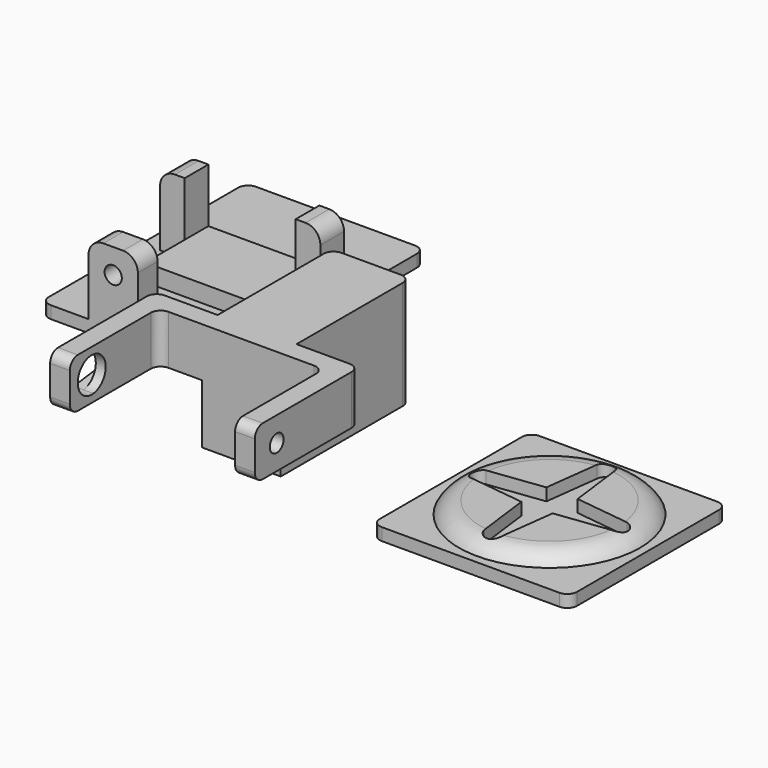
from build123d import *

# Parameters (mm, degrees)
F0_W      = 16
F0_H      = 32.9
F0_R      = 1
F0_W_2    = 12
F0_H_2    = 22.5
F1_DEPTH  = 20
F2_DEPTH  = 4
F3_W      = 16
F3_H      = 32.9
F4_DEPTH  = 2
F6_DEPTH  = 10
F7_R      = 2
F9_DEPTH  = 2
F10_DEPTH = 4
F11_W     = 40
F11_H     = 40
F12_DEPTH = 2.5
F13_W     = 5
F13_H     = 6
F13_W_2   = 10
F13_H_2   = 5
F14_DEPTH = 14.5
F15_DEPTH = 3.5
F16_R     = 3
F17_DEPTH = 12
F18_DEPTH = 3.75
F19_R     = 1.75
F20_DEPTH = 4
F21_R     = 1.75
F22_DEPTH = 5
F23_W     = 40
F23_H     = 40
F24_DEPTH = 2.5
F25_R     = 18.365
F26_DEPTH = 2.5
F28_R     = 2
F29_R     = 2


# Not quite as in the source:
# - a fillet or chamfer that OpenCascade refuses, or shapes differently, is made with other operations: its cross-section is extruded or revolved along the edge and cut away or added


with BuildPart() as f1:
    # F0 (on Top) → F1 (new body)
    with BuildSketch(Plane.XY):
        Rectangle(F0_W, F0_H)
        with Locations((0, -13.85)):
            Circle(F0_R, mode=Mode.SUBTRACT)
        Rectangle(F0_W_2, F0_H_2, mode=Mode.SUBTRACT)
        with Locations((0, 13.85)):
            Circle(F0_R, mode=Mode.SUBTRACT)
        with Locations((0, 13.85)):
            Circle(F0_R)
        with Locations((0, -13.85)):
            Circle(F0_R)
    extrude(amount=F1_DEPTH)

    # F0 (on Top) → F2 (cut)
    with BuildSketch(Plane.XY):
        with Locations((0, 13.85)):
            Circle(F0_R)
        with Locations((0, -13.85)):
            Circle(F0_R)
    extrude(amount=F2_DEPTH, mode=Mode.SUBTRACT)

    # F3 (on face) → F4 (join)
    with BuildSketch(Plane.XY.offset(20)):
        Rectangle(F3_W, F3_H)
    extrude(amount=F4_DEPTH)

    # F5 (on face) → F6 (join)
    with BuildSketch(Plane.XY.offset(22)):
        Polygon((8, -12.45), (8, -16.45), (16.75, -16.45), (16.75, -38.95), (20.75, -38.95), (20.75, -12.45), align=None)
        Polygon((-16.75, -38.95), (-16.75, -16.45), (-8, -16.45), (-8, -12.45), (-20.75, -12.45), (-20.75, -38.95), align=None)
    extrude(amount=-F6_DEPTH)

    # F7
    f7_edges = [f1.edges().sort_by_distance(p)[0] for p in [
        (-20.75, -12.45, 17),
        (20.75, -12.45, 17),
        (18.75, -38.95, 22),
        (18.75, -38.95, 12),
        (-18.75, -38.95, 22),
        (-18.75, -38.95, 12),
        (-16.75, -16.45, 17),
        (16.75, -16.45, 17),
        (-8, 16.45, 11),
        (8, 16.45, 11),
    ]]
    fillet(f7_edges, radius=F7_R)

    # F8 (on face) → F9 (cut)
    with BuildSketch(Plane(origin=(-20.75, 0, 0), x_dir=(0, -1, 0), z_dir=(-1, 0, 0))):
        with BuildLine():
            ThreePointArc((21.11, 17), (20.5076279836, 18.3347630248), (19.1082108626, 18.7661284151))
            ThreePointArc((19.1082108626, 18.7661284151), (17.55, 17), (19.1082108626, 15.2338715849))
            ThreePointArc((19.1082108626, 15.2338715849), (20.5076279836, 15.6652369752), (21.11, 17))
        make_face()
        with BuildLine():
            ThreePointArc((32.9745367412, 13.4925483442), (29.88, 17), (32.9745367412, 20.5074516558))
            Line((32.9745367412, 20.5074516558), (19.1082108626, 18.7661284151))
            ThreePointArc((19.1082108626, 18.7661284151), (20.5076279836, 18.3347630248), (21.11, 17))
            ThreePointArc((21.11, 17), (20.5076279836, 15.6652369752), (19.1082108626, 15.2338715849))
            Line((19.1082108626, 15.2338715849), (32.9745367412, 13.4925483442))
        make_face()
        with BuildLine():
            ThreePointArc((32.9745367412, 13.4925483442), (35.7537162483, 14.3492206222), (36.95, 17))
            ThreePointArc((36.95, 17), (35.7537162483, 19.6507793778), (32.9745367412, 20.5074516558))
            ThreePointArc((32.9745367412, 20.5074516558), (29.88, 17), (32.9745367412, 13.4925483442))
        make_face()
    extrude(amount=-F9_DEPTH, mode=Mode.SUBTRACT)

    # F8 (on face) → F10 (cut, through all)
    with BuildSketch(Plane(origin=(-20.75, 0, 0), x_dir=(0, -1, 0), z_dir=(-1, 0, 0))):
        with BuildLine():
            ThreePointArc((32.9745367412, 13.4925483442), (35.7537162483, 14.3492206222), (36.95, 17))
            ThreePointArc((36.95, 17), (35.7537162483, 19.6507793778), (32.9745367412, 20.5074516558))
            ThreePointArc((32.9745367412, 20.5074516558), (29.88, 17), (32.9745367412, 13.4925483442))
        make_face()
    extrude(amount=-F10_DEPTH, mode=Mode.SUBTRACT)

    # F19 (on face) → F20 (cut, through all)
    with BuildSketch(Plane(origin=(16.75, 0, 0), x_dir=(0, -1, 0), z_dir=(-1, 0, 0))):
        with Locations((33.415, 17)):
            Circle(F19_R)
    extrude(amount=-F20_DEPTH, mode=Mode.SUBTRACT)


with BuildPart() as f12:
    # F11 (on Top) → F12 (new body)
    with BuildSketch(Plane.XY):
        with Locations((-36.1275146902, 22.9365597665)):
            Rectangle(F11_W, F11_H)
    extrude(amount=F12_DEPTH)

    # F13 (on face) → F14 (join)
    with BuildSketch(Plane.XY.offset(2.5)):
        with Locations((-49.8775146902, 31.4365597665)):
            Rectangle(F13_W, F13_H)
        with Locations((-22.3775146902, 31.4365597665)):
            Rectangle(F13_W, F13_H)
        with Locations((-41.4775146902, 5.4365597665)):
            Rectangle(F13_W_2, F13_H_2)
    extrude(amount=F14_DEPTH)

    # F13 (on face) → F15 (join)
    with BuildSketch(Plane.XY.offset(2.5)):
        Polygon((-24.8775146902, 34.4365597665), (-47.3775146902, 34.4365597665), (-47.3775146902, 28.4365597665), (-47.3775146902, 18.4365597665), (-24.8775146902, 18.4365597665), (-24.8775146902, 28.4365597665), align=None)
    extrude(amount=F15_DEPTH)

    # F16
    f16_edges = [f12.edges().sort_by_distance(p)[0] for p in [
        (-52.377515, 31.43656, 17),
        (-19.877515, 31.43656, 17),
        (-46.477515, 5.43656, 17),
        (-36.477515, 5.43656, 17),
    ]]
    fillet(f16_edges, radius=F16_R)

    # F17 (add): a face of the model
    f17_faces = [f12.faces().sort_by_distance(p)[0] for p in [
        (-36.1275146902, 42.9365597665, 1.25),
    ]]
    extrude(f17_faces, amount=F17_DEPTH)

    # F18 (cut, through all): a face of the model
    f18_faces = [f12.faces().sort_by_distance(p)[0] for p in [
        (-16.1275146902, 28.9365597665, 1.25),
    ]]
    extrude(f18_faces, amount=-F18_DEPTH, mode=Mode.SUBTRACT)

    # F21 (on face) → F22 (cut, through all)
    with BuildSketch(Plane(origin=(0, 7.9365597665, 0), x_dir=(-1, 0, 0), z_dir=(0, 1, 0))):
        with Locations((41.4775146902, 12)):
            Circle(F21_R)
    extrude(amount=-F22_DEPTH, mode=Mode.SUBTRACT)

    # F29
    f29_edges = [f12.edges().sort_by_distance(p)[0] for p in [
        (-56.127515, 2.93656, 1.25),
        (-19.877515, 2.93656, 1.25),
        (-19.877515, 54.93656, 1.25),
        (-56.127515, 54.93656, 1.25),
    ]]
    fillet(f29_edges, radius=F29_R)


with BuildPart() as f24:
    # F23 (on Top) → F24 (new body)
    with BuildSketch(Plane.XY):
        with Locations((49.3299849331, 0)):
            Rectangle(F23_W, F23_H)
        with BuildLine():
            ThreePointArc((35.0231957958, -1.7661284151), (33.4649849331, 0), (35.0231957958, 1.7661284151))
            Line((35.0231957958, 1.7661284151), (46.164712816, 3.1652721172))
            Line((46.164712816, 3.1652721172), (47.5638565181, 14.3067891374))
            ThreePointArc((47.5638565181, 14.3067891374), (49.3299849331, 15.865), (51.0961133482, 14.3067891374))
            Line((51.0961133482, 14.3067891374), (52.4952570503, 3.1652721172))
            Line((52.4952570503, 3.1652721172), (63.6367740705, 1.7661284151))
            ThreePointArc((63.6367740705, 1.7661284151), (64.7497479579, 1.1776279836), (65.1949849331, 0))
            ThreePointArc((65.1949849331, 0), (64.7497479579, -1.1776279836), (63.6367740705, -1.7661284151))
            Line((63.6367740705, -1.7661284151), (52.4952570503, -3.1652721172))
            Line((52.4952570503, -3.1652721172), (51.0961133482, -14.3067891374))
            ThreePointArc((51.0961133482, -14.3067891374), (49.3299849331, -15.865), (47.5638565181, -14.3067891374))
            Line((47.5638565181, -14.3067891374), (46.164712816, -3.1652721172))
            Line((46.164712816, -3.1652721172), (35.0231957958, -1.7661284151))
        make_face(mode=Mode.SUBTRACT)
        with BuildLine():
            ThreePointArc((35.0231957958, 1.7661284151), (36.4226129167, 1.3347630248), (37.0249849331, 0))
            ThreePointArc((37.0249849331, 0), (36.4226129167, -1.3347630248), (35.0231957958, -1.7661284151))
            Line((35.0231957958, -1.7661284151), (46.164712816, -3.1652721172))
            Line((46.164712816, -3.1652721172), (47.5638565181, -14.3067891374))
            ThreePointArc((47.5638565181, -14.3067891374), (49.21887368, -12.308471281), (51.1099849331, -14.085))
            ThreePointArc((51.1099849331, -14.085), (51.1065136521, -14.1961112532), (51.0961133482, -14.3067891374))
            Line((51.0961133482, -14.3067891374), (52.4952570503, -3.1652721172))
            Line((52.4952570503, -3.1652721172), (63.6367740705, -1.7661284151))
            ThreePointArc((63.6367740705, -1.7661284151), (61.6349849331, 0), (63.6367740705, 1.7661284151))
            Line((63.6367740705, 1.7661284151), (52.4952570503, 3.1652721172))
            Line((52.4952570503, 3.1652721172), (51.0961133482, 14.3067891374))
            ThreePointArc((51.0961133482, 14.3067891374), (51.1065136521, 14.1961112532), (51.1099849331, 14.085))
            ThreePointArc((51.1099849331, 14.085), (49.21887368, 12.308471281), (47.5638565181, 14.3067891374))
            Line((47.5638565181, 14.3067891374), (46.164712816, 3.1652721172))
            Line((46.164712816, 3.1652721172), (35.0231957958, 1.7661284151))
        make_face()
        with BuildLine():
            ThreePointArc((51.0961133482, 14.3067891374), (49.3299849331, 15.865), (47.5638565181, 14.3067891374))
            ThreePointArc((47.5638565181, 14.3067891374), (49.21887368, 12.308471281), (51.1099849331, 14.085))
            ThreePointArc((51.1099849331, 14.085), (51.1065136521, 14.1961112532), (51.0961133482, 14.3067891374))
        make_face()
        with BuildLine():
            ThreePointArc((35.0231957958, -1.7661284151), (36.4226129167, -1.3347630248), (37.0249849331, 0))
            ThreePointArc((37.0249849331, 0), (36.4226129167, 1.3347630248), (35.0231957958, 1.7661284151))
            ThreePointArc((35.0231957958, 1.7661284151), (33.4649849331, 0), (35.0231957958, -1.7661284151))
        make_face()
        with BuildLine():
            ThreePointArc((51.1099849331, -14.085), (49.21887368, -12.308471281), (47.5638565181, -14.3067891374))
            ThreePointArc((47.5638565181, -14.3067891374), (49.3299849331, -15.865), (51.0961133482, -14.3067891374))
            ThreePointArc((51.0961133482, -14.3067891374), (51.1065136521, -14.1961112532), (51.1099849331, -14.085))
        make_face()
        with BuildLine():
            ThreePointArc((65.1949849331, 0), (64.7497479579, 1.1776279836), (63.6367740705, 1.7661284151))
            ThreePointArc((63.6367740705, 1.7661284151), (61.6349849331, 0), (63.6367740705, -1.7661284151))
            ThreePointArc((63.6367740705, -1.7661284151), (64.7497479579, -1.1776279836), (65.1949849331, 0))
        make_face()
    extrude(amount=-F24_DEPTH)

    # F25 (on face) → F26 (join)
    with BuildSketch(Plane.XY):
        with Locations((49.3299849331, 0)):
            Circle(F25_R)
        with BuildLine():
            Line((46.164712816, -3.1652721172), (35.0231957958, -1.7661284151))
            ThreePointArc((35.0231957958, -1.7661284151), (33.4649849331, 0), (35.0231957958, 1.7661284151))
            Line((35.0231957958, 1.7661284151), (46.164712816, 3.1652721172))
            Line((46.164712816, 3.1652721172), (47.5638565181, 14.3067891374))
            ThreePointArc((47.5638565181, 14.3067891374), (49.3299849331, 15.865), (51.0961133482, 14.3067891374))
            Line((51.0961133482, 14.3067891374), (52.4952570503, 3.1652721172))
            Line((52.4952570503, 3.1652721172), (63.6367740705, 1.7661284151))
            ThreePointArc((63.6367740705, 1.7661284151), (64.7497479579, 1.1776279836), (65.1949849331, 0))
            ThreePointArc((65.1949849331, 0), (64.7497479579, -1.1776279836), (63.6367740705, -1.7661284151))
            Line((63.6367740705, -1.7661284151), (52.4952570503, -3.1652721172))
            Line((52.4952570503, -3.1652721172), (51.0961133482, -14.3067891374))
            ThreePointArc((51.0961133482, -14.3067891374), (49.3299849331, -15.865), (47.5638565181, -14.3067891374))
            Line((47.5638565181, -14.3067891374), (46.164712816, -3.1652721172))
        make_face(mode=Mode.SUBTRACT)
    extrude(amount=F26_DEPTH)

    # F27: fillet of radius 5 on 1 edges, made by hand

    # F27_s1 → F27_t2 (revolve, cut)
    with BuildSketch(Plane.XZ):
        with BuildLine():
            ThreePointArc((67.6949849331, 0), (65.8648579142, 1.8301270189), (63.3648579142, 2.5))
            Line((63.3648579142, 2.5), (67.6949849331, 2.5))
            Line((67.6949849331, 2.5), (67.6949849331, 0))
        make_face()
    revolve(axis=Axis((49.3299849331, 0, 2.5), (0, 0, 1)), mode=Mode.SUBTRACT)

    # F28
    f28_edges = [f24.edges().sort_by_distance(p)[0] for p in [
        (29.329985, 20, -1.25),
        (69.329985, 20, -1.25),
        (69.329985, -20, -1.25),
        (29.329985, -20, -1.25),
    ]]
    fillet(f28_edges, radius=F28_R)


solid = Compound([f1.part, f12.part, f24.part])
